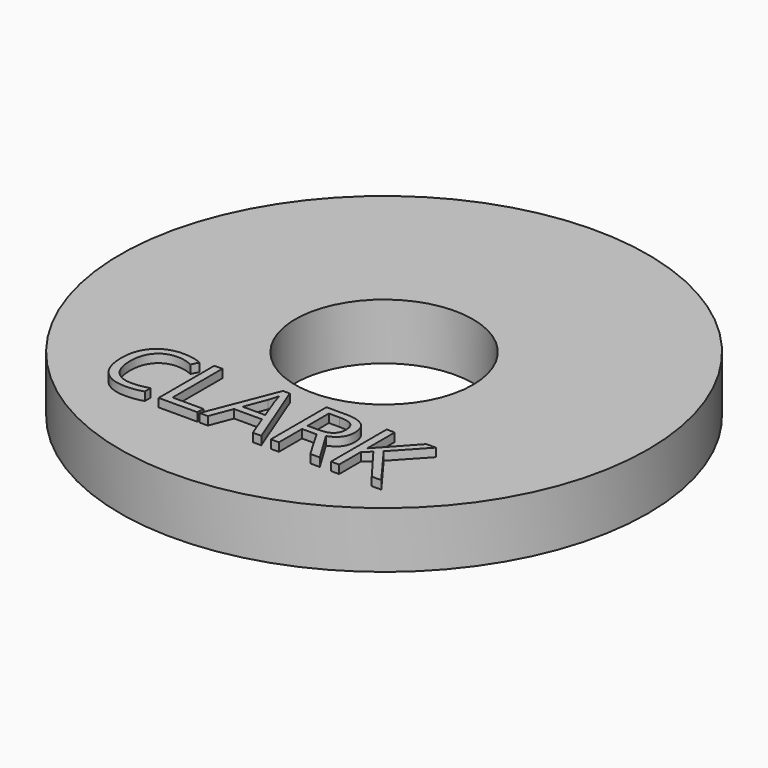
from build123d import *

# Parameters (mm, degrees)
F0_R         = 32.6825151338
F0_R_2       = 11
F1_DEPTH     = 6.96
F2_TEXT_SIZE = 12.0597270628
F3_DEPTH     = 8


# Not quite as in the source:
# - Text() gives the source's letters only with a copy of the font that has no kerning and outlines rounded to 1/6400 em; it was checked with that copy


with BuildPart() as f1:
    # F0 (on Top) → F1 (new body)
    with BuildSketch(Plane.XY):
        Circle(F0_R)
        Circle(F0_R_2, mode=Mode.SUBTRACT)
    extrude(amount=F1_DEPTH)

    # F2 (on Top) → F3 (join)
    with BuildSketch(Plane.XY):
        with Locations((-18.5691531782, -22.6722843945)):
            Text('CLARK', F2_TEXT_SIZE, font='Open Sans', text_align=(TextAlign.LEFT, TextAlign.BOTTOM))
    extrude(amount=F3_DEPTH)


solid = f1.part
